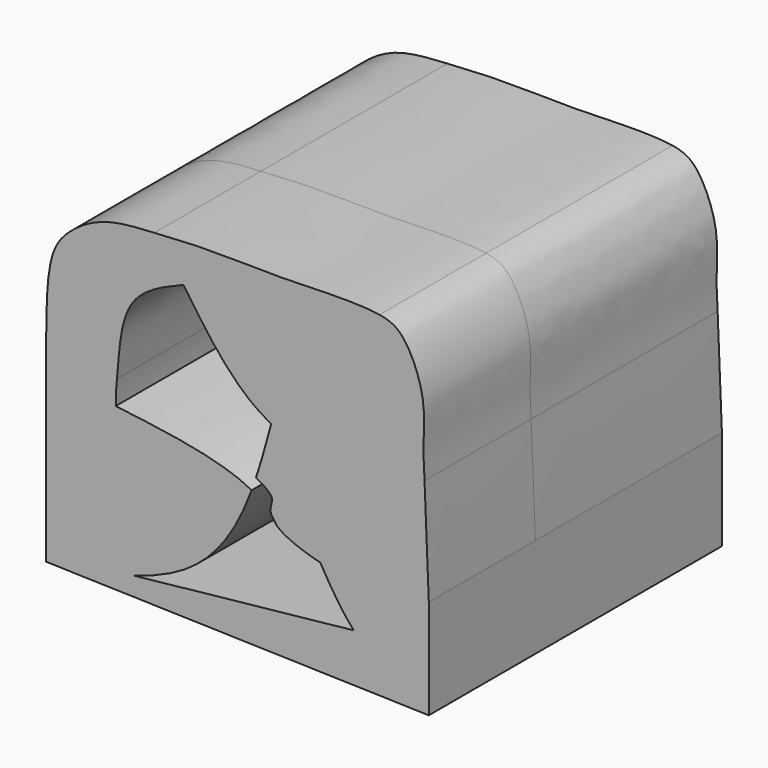
from build123d import *

# Parameters (mm, degrees)
F1_DEPTH = 65.786
F2_DEPTH = 37.592


with BuildPart() as f1:
    # F0 (on Front) → F1 (new body)
    with BuildSketch(Plane.XZ):
        with BuildLine():
            add(Edge.make_bspline(
                [(-63.5240077972, 0), (-56.800894212, -1.0775298684), (-50.0777806268, -2.1550597368), (-43.5278602812, -2.9725744292)],
                knots=[0, 0, 0, 0, 0.1517041989, 0.1517041989, 0.1517041989, 0.1517041989], degree=3))
            add(Edge.make_bspline(
                [(-63.5240077972, 0), (-63.5240077972, -14.8315681088), (-63.5240077972, -38.8086731136), (-63.5240077972, -50.459096132), (-63.5240077972, -54.9028925598)],
                knots=[0, 0, 0, 0, 0.6185720964, 1, 1, 1, 1], degree=3))
            add(Edge.make_bspline(
                [(-38.6864171805, -50.2711780887), (-50.9512119334, -53.9625100963), (-63.4495334183, -54.869292182), (-63.5240077972, -54.9028925598)],
                knots=[0.6463482271, 0.6463482271, 0.6463482271, 0.6463482271, 0.9807009616, 0.9807009616, 0.9807009616, 0.9807009616], degree=3))
            add(Edge.make_bspline(
                [(-5.5222542955, -18.2656030645), (-9.6177271454, -29.334625985), (-17.4503709129, -42.4788636865), (-34.347240688, -48.9652172963), (-38.6864171805, -50.2711780887)],
                knots=[0.1825956876, 0.1825956876, 0.1825956876, 0.1825956876, 0.5280571708, 0.6463482271, 0.6463482271, 0.6463482271, 0.6463482271], degree=3))
            add(Edge.make_bspline(
                [(-5.5222542955, -18.2656030645), (-14.3615559782, -13.5084226746), (-29.1116867734, -11.6697593601), (-43.8618175685, -9.8310960457)],
                knots=[0.536277576, 0.536277576, 0.536277576, 0.536277576, 1, 1, 1, 1], degree=3))
            add(Edge.make_bspline(
                [(-43.5278602812, -2.9725744292), (-43.7574319507, -5.4534811837), (-43.9319764374, -7.5593468165), (-43.8618175685, -9.8310960457)],
                knots=[0.364256955, 0.364256955, 0.364256955, 0.364256955, 0.454666135, 0.454666135, 0.454666135, 0.454666135], degree=3))
        make_face()
        with BuildLine():
            add(Edge.make_bspline(
                [(30.5520221591, 37.0556712151), (34.0105628024, 36.4734212431), (38.1054530927, 33.9530063414), (43.8199870431, 20.7878269574), (42.6933877746, 8.671351149), (43.0629264411, 3.7159273768), (43.2568266988, 0)],
                knots=[0.624432363, 0.624432363, 0.624432363, 0.624432363, 0.6822121522, 0.7571029707, 0.827315679, 0.8883884684, 0.8883884684, 0.8883884684, 0.8883884684], degree=3))
            add(Edge.make_bspline(
                [(13.8594305388, 10.8592628278), (20.3273577037, 18.2346283086), (25.4396899314, 27.6451497618), (30.5520221591, 37.0556712151)],
                knots=[0.7125110381, 0.7125110381, 0.7125110381, 0.7125110381, 1, 1, 1, 1], degree=3))
            add(Edge.make_bspline(
                [(13.8594305388, 10.8592628278), (17.5604882015, 6.5582793426), (21.2565043667, 2.2290147137), (23.9242081779, -3.1279210775)],
                knots=[0, 0, 0, 0, 0.1597565298, 0.1597565298, 0.1597565298, 0.1597565298], degree=3))
            add(Edge.make_bspline(
                [(43.2568266988, 0), (36.7271959027, -1.2648272998), (30.1975651067, -2.5296545995), (23.9242081779, -3.1279210775)],
                knots=[0, 0, 0, 0, 0.1699095992, 0.1699095992, 0.1699095992, 0.1699095992], degree=3))
        make_face()
        with BuildLine():
            add(Edge.make_bspline(
                [(-32.9719856381, 36.7531776428), (-29.0195790904, 36.9869114892), (-21.8300737753, 37.5502432541), (-4.4364884364, 37.370612376), (5.8593016392, 37.152577587), (24.5712134077, 38.0625484176), (30.5520221591, 37.0556712151)],
                knots=[0.3023646182, 0.3023646182, 0.3023646182, 0.3023646182, 0.3717078691, 0.4543133623, 0.524514535, 0.624432363, 0.624432363, 0.624432363, 0.624432363], degree=3))
            add(Edge.make_bspline(
                [(-24.8046126217, 26.4683365822), (-28.1533623745, 31.1750804496), (-30.5626740063, 33.9641290462), (-32.9719856381, 36.7531776428)],
                knots=[0.7766252382, 0.7766252382, 0.7766252382, 0.7766252382, 1, 1, 1, 1], degree=3))
            add(Edge.make_bspline(
                [(0, 0), (-11.0790603922, 5.5270215272), (-19.2392119365, 18.6460394629), (-24.8046126217, 26.4683365822)],
                knots=[0.4053911526, 0.4053911526, 0.4053911526, 0.4053911526, 0.7766252382, 0.7766252382, 0.7766252382, 0.7766252382], degree=3))
            add(Edge.make_bspline(
                [(0, 0), (-1.3505629892, 10.3087183451), (-3.9277431014, 29.9164532393), (8.1573168133, 16.967743401), (13.8594305388, 10.8592628278)],
                knots=[0, 0, 0, 0, 0.5264929724, 1, 1, 1, 1], degree=3))
            add(Edge.make_bspline(
                [(13.8594305388, 10.8592628278), (20.3273577037, 18.2346283086), (25.4396899314, 27.6451497618), (30.5520221591, 37.0556712151)],
                knots=[0.7125110381, 0.7125110381, 0.7125110381, 0.7125110381, 1, 1, 1, 1], degree=3))
        make_face()
        with BuildLine():
            add(Edge.make_bspline(
                [(0, 0), (-1.3505629892, 10.3087183451), (-3.9277431014, 29.9164532393), (8.1573168133, 16.967743401), (13.8594305388, 10.8592628278)],
                knots=[0, 0, 0, 0, 0.5264929724, 1, 1, 1, 1], degree=3))
            add(Edge.make_bspline(
                [(0, 0), (5.3503012941, 2.523067269), (9.8635631765, 6.302782605), (13.8594305388, 10.8592628278)],
                knots=[0.5349011592, 0.5349011592, 0.5349011592, 0.5349011592, 0.7125110381, 0.7125110381, 0.7125110381, 0.7125110381], degree=3))
        make_face()
        with BuildLine():
            add(Edge.make_bspline(
                [(0, 0), (5.3503012941, 2.523067269), (9.8635631765, 6.302782605), (13.8594305388, 10.8592628278)],
                knots=[0.5349011592, 0.5349011592, 0.5349011592, 0.5349011592, 0.7125110381, 0.7125110381, 0.7125110381, 0.7125110381], degree=3))
            add(Edge.make_bspline(
                [(23.9242081779, -3.1279210775), (15.2298210333, -3.9570721102), (7.0276799799, -3.5059054793), (0, 0)],
                knots=[0.1699095992, 0.1699095992, 0.1699095992, 0.1699095992, 0.4053911526, 0.4053911526, 0.4053911526, 0.4053911526], degree=3))
            add(Edge.make_bspline(
                [(13.8594305388, 10.8592628278), (17.5604882015, 6.5582793426), (21.2565043667, 2.2290147137), (23.9242081779, -3.1279210775)],
                knots=[0, 0, 0, 0, 0.1597565298, 0.1597565298, 0.1597565298, 0.1597565298], degree=3))
        make_face()
        with BuildLine():
            add(Edge.make_bspline(
                [(23.9242081779, -3.1279210775), (15.2298210333, -3.9570721102), (7.0276799799, -3.5059054793), (0, 0)],
                knots=[0.1699095992, 0.1699095992, 0.1699095992, 0.1699095992, 0.4053911526, 0.4053911526, 0.4053911526, 0.4053911526], degree=3))
            add(Edge.make_bspline(
                [(0, 0), (4.4728324678, -10.5492547403), (8.9456649356, -21.0985094806), (13.8594305239, -29.9524251855)],
                knots=[0, 0, 0, 0, 0.3636574997, 0.3636574997, 0.3636574997, 0.3636574997], degree=3))
            add(Edge.make_bspline(
                [(23.9242081779, -3.1279210775), (26.6204532145, -8.5421696451), (29.5766972297, -20.153001473), (21.810722237, -31.3197789457), (16.7217291382, -30.6506424008), (13.8594305388, -29.9524252122)],
                knots=[0.1597565298, 0.1597565298, 0.1597565298, 0.1597565298, 0.3212222626, 0.4497849367, 0.5538859787, 0.5538859787, 0.5538859787, 0.5538859787], degree=3))
        make_face()
        with BuildLine():
            add(Edge.make_bspline(
                [(0, 0), (4.4728324678, -10.5492547403), (8.9456649356, -21.0985094806), (13.8594305239, -29.9524251855)],
                knots=[0, 0, 0, 0, 0.3636574997, 0.3636574997, 0.3636574997, 0.3636574997], degree=3))
            add(Edge.make_bspline(
                [(0, 0), (-1.3539150879, -5.0062615134), (-2.7078301758, -10.0125230268), (-4.316626864, -14.8315680972)],
                knots=[0, 0, 0, 0, 0.1472607818, 0.1472607818, 0.1472607818, 0.1472607818], degree=3))
            add(Edge.make_bspline(
                [(0, -22.5358977914), (-0.2635636531, -21.7047236316), (-0.1272346241, -20.0889351399), (0.9365763808, -17.7222891685), (-3.3889358906, -15.1105107507), (-4.3166268678, -14.8315681088)],
                knots=[0.766461406, 0.766461406, 0.766461406, 0.766461406, 0.8263295038, 0.8829450572, 0.9717632395, 0.9717632395, 0.9717632395, 0.9717632395], degree=3))
            add(Edge.make_bspline(
                [(1.488152394, -24.70578484), (1.0691570646, -23.9444424302), (0.5763910158, -23.2195248774), (0, -22.5358977914)],
                knots=[0.3684861738, 0.3684861738, 0.3684861738, 0.3684861738, 0.4177083301, 0.4177083301, 0.4177083301, 0.4177083301], degree=3))
            add(Edge.make_bspline(
                [(13.8594305388, -29.9524252122), (10.2585116388, -29.0740320666), (4.7263466302, -27.2293564363), (1.9133329744, -25.0987912775), (1.488152394, -24.70578484)],
                knots=[0.5538859787, 0.5538859787, 0.5538859787, 0.5538859787, 0.6848504454, 0.7139186659, 0.7139186659, 0.7139186659, 0.7139186659], degree=3))
        make_face()
        with BuildLine():
            add(Edge.make_bspline(
                [(43.2568266988, 0), (43.6111826237, -6.7909186818), (44.038995531, -18.2933515925), (44.4668084383, -29.7957845032)],
                knots=[0.8883884684, 0.8883884684, 0.8883884684, 0.8883884684, 1, 1, 1, 1], degree=3))
            add(Edge.make_bspline(
                [(43.2568266988, 0), (36.7271959027, -1.2648272998), (30.1975651067, -2.5296545995), (23.9242081779, -3.1279210775)],
                knots=[0, 0, 0, 0, 0.1699095992, 0.1699095992, 0.1699095992, 0.1699095992], degree=3))
            add(Edge.make_bspline(
                [(23.9242081779, -3.1279210775), (26.6204532145, -8.5421696451), (29.5766972297, -20.153001473), (21.810722237, -31.3197789457), (16.7217291382, -30.6506424008), (13.8594305388, -29.9524252122)],
                knots=[0.1597565298, 0.1597565298, 0.1597565298, 0.1597565298, 0.3212222626, 0.4497849367, 0.5538859787, 0.5538859787, 0.5538859787, 0.5538859787], degree=3))
            add(Edge.make_bspline(
                [(13.8594305239, -29.9524251855), (16.8125078822, -35.2734559774), (19.9248403959, -39.9821683267), (23.2921373099, -43.7105707824)],
                knots=[0.3636574997, 0.3636574997, 0.3636574997, 0.3636574997, 0.58220857, 0.58220857, 0.58220857, 0.58220857], degree=3))
            add(Edge.make_bspline(
                [(23.2921373099, -43.7105707824), (29.7292039017, -50.8379419353), (37.09800617, -54.3828925593), (44.4668084383, -57.9278431833)],
                knots=[0.58220857, 0.58220857, 0.58220857, 0.58220857, 1, 1, 1, 1], degree=3))
            add(Edge.make_bspline(
                [(44.4668084383, -29.7957845032), (44.4668084383, -39.1731373966), (44.4668084383, -48.5504902899), (44.4668084383, -57.9278431833)],
                knots=[0, 0, 0, 0, 28.1320586801, 28.1320586801, 28.1320586801, 28.1320586801], degree=3))
        make_face()
        with BuildLine():
            add(Edge.make_bspline(
                [(-63.5240077972, 0), (-63.4541196718, 8.3226000217), (-63.3391779129, 22.0103943304), (-56.9568040639, 29.8479836401), (-47.1288987651, 36.0612304876), (-37.335938301, 36.4951061542), (-32.9719856381, 36.7531776428)],
                knots=[0, 0, 0, 0, 0.095878703, 0.1576872566, 0.2258009701, 0.3023646182, 0.3023646182, 0.3023646182, 0.3023646182], degree=3))
            add(Edge.make_bspline(
                [(-63.5240077972, 0), (-56.800894212, -1.0775298684), (-50.0777806268, -2.1550597368), (-43.5278602812, -2.9725744292)],
                knots=[0, 0, 0, 0, 0.1517041989, 0.1517041989, 0.1517041989, 0.1517041989], degree=3))
            add(Edge.make_bspline(
                [(-24.8046126217, 26.4683365822), (-30.5304064505, 24.1328709252), (-42.0237334945, 19.4449147399), (-42.8894476385, 3.7449684225), (-43.4419108928, -2.043747198), (-43.5278602812, -2.9725744292)],
                knots=[0, 0, 0, 0, 0.1646043618, 0.330408642, 0.364256955, 0.364256955, 0.364256955, 0.364256955], degree=3))
            add(Edge.make_bspline(
                [(-24.8046126217, 26.4683365822), (-28.1533623745, 31.1750804496), (-30.5626740063, 33.9641290462), (-32.9719856381, 36.7531776428)],
                knots=[0.7766252382, 0.7766252382, 0.7766252382, 0.7766252382, 1, 1, 1, 1], degree=3))
        make_face()
        with BuildLine():
            add(Edge.make_bspline(
                [(-38.6864171805, -50.2711780887), (-50.9512119334, -53.9625100963), (-63.4495334183, -54.869292182), (-63.5240077972, -54.9028925598)],
                knots=[0.6463482271, 0.6463482271, 0.6463482271, 0.6463482271, 0.9807009616, 0.9807009616, 0.9807009616, 0.9807009616], degree=3))
            add(Edge.make_bspline(
                [(-63.5240077972, -54.9028925598), (-63.5283065026, -54.9048319935), (-63.4912130872, -54.9038622766), (-63.4541196718, -54.9028925598)],
                knots=[0.9807009616, 0.9807009616, 0.9807009616, 0.9807009616, 1, 1, 1, 1], degree=3))
            add(Edge.make_bspline(
                [(-63.4541196718, -54.9028925598), (-27.4804769685, -55.9112094343), (8.4931657349, -56.9195263088), (44.4668084383, -57.9278431833)],
                knots=[0, 0, 0, 0, 107.9633134469, 107.9633134469, 107.9633134469, 107.9633134469], degree=3))
            add(Edge.make_bspline(
                [(23.2921373099, -43.7105707824), (29.7292039017, -50.8379419353), (37.09800617, -54.3828925593), (44.4668084383, -57.9278431833)],
                knots=[0.58220857, 0.58220857, 0.58220857, 0.58220857, 1, 1, 1, 1], degree=3))
            add(Edge.make_bspline(
                [(-38.6864171805, -50.2711780887), (-18.0238019664, -48.094599226), (2.6295220958, -45.8871496451), (23.2921373099, -43.7105707824)],
                knots=[0, 0, 0, 0, 62.3248167662, 62.3248167662, 62.3248167662, 62.3248167662], degree=3))
        make_face()
    extrude(amount=-F1_DEPTH)

    # F0 (on Front) + F1_face (on face) + F1_face1 (on face) → F2 (join)
    with BuildSketch(Plane.XZ):
        with BuildLine():
            add(Edge.make_bspline(
                [(-63.5240077972, 0), (-63.4541196718, 8.3226000217), (-63.3391779129, 22.0103943304), (-56.9568040639, 29.8479836401), (-47.1288987651, 36.0612304876), (-37.335938301, 36.4951061542), (-32.9719856381, 36.7531776428)],
                knots=[0, 0, 0, 0, 0.095878703, 0.1576872566, 0.2258009701, 0.3023646182, 0.3023646182, 0.3023646182, 0.3023646182], degree=3))
            add(Edge.make_bspline(
                [(-63.5240077972, 0), (-56.800894212, -1.0775298684), (-50.0777806268, -2.1550597368), (-43.5278602812, -2.9725744292)],
                knots=[0, 0, 0, 0, 0.1517041989, 0.1517041989, 0.1517041989, 0.1517041989], degree=3))
            add(Edge.make_bspline(
                [(-24.8046126217, 26.4683365822), (-30.5304064505, 24.1328709252), (-42.0237334945, 19.4449147399), (-42.8894476385, 3.7449684225), (-43.4419108928, -2.043747198), (-43.5278602812, -2.9725744292)],
                knots=[0, 0, 0, 0, 0.1646043618, 0.330408642, 0.364256955, 0.364256955, 0.364256955, 0.364256955], degree=3))
            add(Edge.make_bspline(
                [(-24.8046126217, 26.4683365822), (-28.1533623745, 31.1750804496), (-30.5626740063, 33.9641290462), (-32.9719856381, 36.7531776428)],
                knots=[0.7766252382, 0.7766252382, 0.7766252382, 0.7766252382, 1, 1, 1, 1], degree=3))
        make_face()
        with BuildLine():
            add(Edge.make_bspline(
                [(30.5520221591, 37.0556712151), (34.0105628024, 36.4734212431), (38.1054530927, 33.9530063414), (43.8199870431, 20.7878269574), (42.6933877746, 8.671351149), (43.0629264411, 3.7159273768), (43.2568266988, 0)],
                knots=[0.624432363, 0.624432363, 0.624432363, 0.624432363, 0.6822121522, 0.7571029707, 0.827315679, 0.8883884684, 0.8883884684, 0.8883884684, 0.8883884684], degree=3))
            add(Edge.make_bspline(
                [(13.8594305388, 10.8592628278), (20.3273577037, 18.2346283086), (25.4396899314, 27.6451497618), (30.5520221591, 37.0556712151)],
                knots=[0.7125110381, 0.7125110381, 0.7125110381, 0.7125110381, 1, 1, 1, 1], degree=3))
            add(Edge.make_bspline(
                [(13.8594305388, 10.8592628278), (17.5604882015, 6.5582793426), (21.2565043667, 2.2290147137), (23.9242081779, -3.1279210775)],
                knots=[0, 0, 0, 0, 0.1597565298, 0.1597565298, 0.1597565298, 0.1597565298], degree=3))
            add(Edge.make_bspline(
                [(43.2568266988, 0), (36.7271959027, -1.2648272998), (30.1975651067, -2.5296545995), (23.9242081779, -3.1279210775)],
                knots=[0, 0, 0, 0, 0.1699095992, 0.1699095992, 0.1699095992, 0.1699095992], degree=3))
        make_face()
        with BuildLine():
            add(Edge.make_bspline(
                [(-38.6864171805, -50.2711780887), (-50.9512119334, -53.9625100963), (-63.4495334183, -54.869292182), (-63.5240077972, -54.9028925598)],
                knots=[0.6463482271, 0.6463482271, 0.6463482271, 0.6463482271, 0.9807009616, 0.9807009616, 0.9807009616, 0.9807009616], degree=3))
            add(Edge.make_bspline(
                [(-63.5240077972, -54.9028925598), (-63.5283065026, -54.9048319935), (-63.4912130872, -54.9038622766), (-63.4541196718, -54.9028925598)],
                knots=[0.9807009616, 0.9807009616, 0.9807009616, 0.9807009616, 1, 1, 1, 1], degree=3))
            add(Edge.make_bspline(
                [(-63.4541196718, -54.9028925598), (-27.4804769685, -55.9112094343), (8.4931657349, -56.9195263088), (44.4668084383, -57.9278431833)],
                knots=[0, 0, 0, 0, 107.9633134469, 107.9633134469, 107.9633134469, 107.9633134469], degree=3))
            add(Edge.make_bspline(
                [(23.2921373099, -43.7105707824), (29.7292039017, -50.8379419353), (37.09800617, -54.3828925593), (44.4668084383, -57.9278431833)],
                knots=[0.58220857, 0.58220857, 0.58220857, 0.58220857, 1, 1, 1, 1], degree=3))
            add(Edge.make_bspline(
                [(-38.6864171805, -50.2711780887), (-18.0238019664, -48.094599226), (2.6295220958, -45.8871496451), (23.2921373099, -43.7105707824)],
                knots=[0, 0, 0, 0, 62.3248167662, 62.3248167662, 62.3248167662, 62.3248167662], degree=3))
        make_face()
        with BuildLine():
            add(Edge.make_bspline(
                [(-32.9719856381, 36.7531776428), (-29.0195790904, 36.9869114892), (-21.8300737753, 37.5502432541), (-4.4364884364, 37.370612376), (5.8593016392, 37.152577587), (24.5712134077, 38.0625484176), (30.5520221591, 37.0556712151)],
                knots=[0.3023646182, 0.3023646182, 0.3023646182, 0.3023646182, 0.3717078691, 0.4543133623, 0.524514535, 0.624432363, 0.624432363, 0.624432363, 0.624432363], degree=3))
            add(Edge.make_bspline(
                [(-24.8046126217, 26.4683365822), (-28.1533623745, 31.1750804496), (-30.5626740063, 33.9641290462), (-32.9719856381, 36.7531776428)],
                knots=[0.7766252382, 0.7766252382, 0.7766252382, 0.7766252382, 1, 1, 1, 1], degree=3))
            add(Edge.make_bspline(
                [(0, 0), (-11.0790603922, 5.5270215272), (-19.2392119365, 18.6460394629), (-24.8046126217, 26.4683365822)],
                knots=[0.4053911526, 0.4053911526, 0.4053911526, 0.4053911526, 0.7766252382, 0.7766252382, 0.7766252382, 0.7766252382], degree=3))
            add(Edge.make_bspline(
                [(0, 0), (-1.3505629892, 10.3087183451), (-3.9277431014, 29.9164532393), (8.1573168133, 16.967743401), (13.8594305388, 10.8592628278)],
                knots=[0, 0, 0, 0, 0.5264929724, 1, 1, 1, 1], degree=3))
            add(Edge.make_bspline(
                [(13.8594305388, 10.8592628278), (20.3273577037, 18.2346283086), (25.4396899314, 27.6451497618), (30.5520221591, 37.0556712151)],
                knots=[0.7125110381, 0.7125110381, 0.7125110381, 0.7125110381, 1, 1, 1, 1], degree=3))
        make_face()
        with BuildLine():
            add(Edge.make_bspline(
                [(43.2568266988, 0), (43.6111826237, -6.7909186818), (44.038995531, -18.2933515925), (44.4668084383, -29.7957845032)],
                knots=[0.8883884684, 0.8883884684, 0.8883884684, 0.8883884684, 1, 1, 1, 1], degree=3))
            add(Edge.make_bspline(
                [(43.2568266988, 0), (36.7271959027, -1.2648272998), (30.1975651067, -2.5296545995), (23.9242081779, -3.1279210775)],
                knots=[0, 0, 0, 0, 0.1699095992, 0.1699095992, 0.1699095992, 0.1699095992], degree=3))
            add(Edge.make_bspline(
                [(23.9242081779, -3.1279210775), (26.6204532145, -8.5421696451), (29.5766972297, -20.153001473), (21.810722237, -31.3197789457), (16.7217291382, -30.6506424008), (13.8594305388, -29.9524252122)],
                knots=[0.1597565298, 0.1597565298, 0.1597565298, 0.1597565298, 0.3212222626, 0.4497849367, 0.5538859787, 0.5538859787, 0.5538859787, 0.5538859787], degree=3))
            add(Edge.make_bspline(
                [(13.8594305239, -29.9524251855), (16.8125078822, -35.2734559774), (19.9248403959, -39.9821683267), (23.2921373099, -43.7105707824)],
                knots=[0.3636574997, 0.3636574997, 0.3636574997, 0.3636574997, 0.58220857, 0.58220857, 0.58220857, 0.58220857], degree=3))
            add(Edge.make_bspline(
                [(23.2921373099, -43.7105707824), (29.7292039017, -50.8379419353), (37.09800617, -54.3828925593), (44.4668084383, -57.9278431833)],
                knots=[0.58220857, 0.58220857, 0.58220857, 0.58220857, 1, 1, 1, 1], degree=3))
            add(Edge.make_bspline(
                [(44.4668084383, -29.7957845032), (44.4668084383, -39.1731373966), (44.4668084383, -48.5504902899), (44.4668084383, -57.9278431833)],
                knots=[0, 0, 0, 0, 28.1320586801, 28.1320586801, 28.1320586801, 28.1320586801], degree=3))
        make_face()
        with BuildLine():
            add(Edge.make_bspline(
                [(-63.5240077972, 0), (-56.800894212, -1.0775298684), (-50.0777806268, -2.1550597368), (-43.5278602812, -2.9725744292)],
                knots=[0, 0, 0, 0, 0.1517041989, 0.1517041989, 0.1517041989, 0.1517041989], degree=3))
            add(Edge.make_bspline(
                [(-63.5240077972, 0), (-63.5240077972, -14.8315681088), (-63.5240077972, -38.8086731136), (-63.5240077972, -50.459096132), (-63.5240077972, -54.9028925598)],
                knots=[0, 0, 0, 0, 0.6185720964, 1, 1, 1, 1], degree=3))
            add(Edge.make_bspline(
                [(-38.6864171805, -50.2711780887), (-50.9512119334, -53.9625100963), (-63.4495334183, -54.869292182), (-63.5240077972, -54.9028925598)],
                knots=[0.6463482271, 0.6463482271, 0.6463482271, 0.6463482271, 0.9807009616, 0.9807009616, 0.9807009616, 0.9807009616], degree=3))
            add(Edge.make_bspline(
                [(-5.5222542955, -18.2656030645), (-9.6177271454, -29.334625985), (-17.4503709129, -42.4788636865), (-34.347240688, -48.9652172963), (-38.6864171805, -50.2711780887)],
                knots=[0.1825956876, 0.1825956876, 0.1825956876, 0.1825956876, 0.5280571708, 0.6463482271, 0.6463482271, 0.6463482271, 0.6463482271], degree=3))
            add(Edge.make_bspline(
                [(-5.5222542955, -18.2656030645), (-14.3615559782, -13.5084226746), (-29.1116867734, -11.6697593601), (-43.8618175685, -9.8310960457)],
                knots=[0.536277576, 0.536277576, 0.536277576, 0.536277576, 1, 1, 1, 1], degree=3))
            add(Edge.make_bspline(
                [(-43.5278602812, -2.9725744292), (-43.7574319507, -5.4534811837), (-43.9319764374, -7.5593468165), (-43.8618175685, -9.8310960457)],
                knots=[0.364256955, 0.364256955, 0.364256955, 0.364256955, 0.454666135, 0.454666135, 0.454666135, 0.454666135], degree=3))
        make_face()
    with BuildSketch(Plane(origin=(-7.6226899771, 0, -10.0369627759), x_dir=(1, 0, 0), z_dir=(0, -1, 0))):
        with BuildLine():
            add(Edge.make_bspline(
                [(-55.9013178202, 10.0369627759), (-55.9013178202, -4.7946053329), (-55.9013178202, -28.7717103377), (-55.9013178202, -40.4221333561), (-55.9013178202, -44.8659297839)],
                knots=[0, 0, 0, 0, 0.6185720964, 1, 1, 1, 1], degree=3))
            add(Edge.make_bspline(
                [(-55.9013178202, -44.8659297839), (-55.9056165255, -44.8678692176), (-55.8685231102, -44.8668995008), (-55.8314296948, -44.8659297839)],
                knots=[0.9807009616, 0.9807009616, 0.9807009616, 0.9807009616, 1, 1, 1, 1], degree=3))
            add(Edge.make_bspline(
                [(-55.8314296948, -44.8659297839), (-19.8577869914, -45.8742466584), (16.115855712, -46.8825635329), (52.0894984154, -47.8908804074)],
                knots=[0, 0, 0, 0, 107.9633134469, 107.9633134469, 107.9633134469, 107.9633134469], degree=3))
            add(Edge.make_bspline(
                [(52.0894984154, -19.7588217273), (52.0894984154, -29.1361746207), (52.0894984154, -38.513527514), (52.0894984154, -47.8908804074)],
                knots=[0, 0, 0, 0, 28.1320586801, 28.1320586801, 28.1320586801, 28.1320586801], degree=3))
            add(Edge.make_bspline(
                [(52.0894984154, -19.7588217273), (51.6616855081, -8.2563888166), (50.9997773673, 9.5400681217), (50.3160777517, 18.7083139249), (51.4426770202, 30.8247897333), (45.7281430698, 43.9899691172), (38.5492799946, 48.4085767452), (13.4819916163, 47.1895403629), (3.1862015407, 47.4075751518), (-14.2073837983, 47.58720603), (-25.0195235656, 46.7400237121), (-39.506208788, 46.0981932634), (-49.3341140868, 39.884946416), (-55.7164879359, 32.0473571063), (-55.8314296948, 18.3595627976), (-55.9013178202, 10.0369627759)],
                knots=[0.8883884684, 0.8883884684, 0.8883884684, 0.8883884684, 1, 1.0610727893, 1.1312854977, 1.2061763162, 1.2639561054, 1.3638739333, 1.434075106, 1.5166805993, 1.5860238501, 1.6625874983, 1.7307012118, 1.7925097654, 1.8883884684, 1.8883884684, 1.8883884684, 1.8883884684], degree=3))
        make_face()
        with BuildLine():
            add(Edge.make_bspline(
                [(-31.0637272034, -40.2342153128), (-26.7245507109, -38.9282545204), (-9.8276809358, -32.4419009106), (-1.9950371683, -19.2976632091), (2.1004356815, -8.2286402886)],
                knots=[0.9807009616, 0.9807009616, 0.9807009616, 0.9807009616, 1.0989920179, 1.4444535011, 1.4444535011, 1.4444535011, 1.4444535011], degree=3))
            add(Edge.make_bspline(
                [(2.1004356815, -8.2286402886), (-6.7388660012, -3.4714598987), (-21.4889967963, -1.6327965842), (-36.2391275915, 0.2058667302)],
                knots=[0.536277576, 0.536277576, 0.536277576, 0.536277576, 1, 1, 1, 1], degree=3))
            add(Edge.make_bspline(
                [(-36.2391275915, 0.2058667302), (-36.3355532548, 3.3281366583), (-35.4816293471, 9.8851784973), (-34.4010435174, 29.4818775158), (-22.9077164735, 34.1698337011), (-17.1819226446, 36.5052993581)],
                knots=[0.364256955, 0.364256955, 0.364256955, 0.364256955, 0.488514448, 0.6543187282, 0.81892309, 0.81892309, 0.81892309, 0.81892309], degree=3))
            add(Edge.make_bspline(
                [(-17.1819226446, 36.5052993581), (-11.6165219594, 28.6830022388), (-3.4563704151, 15.563984303), (7.6226899771, 10.0369627759)],
                knots=[1, 1, 1, 1, 1.3712340856, 1.3712340856, 1.3712340856, 1.3712340856], degree=3))
            add(Edge.make_bspline(
                [(7.6226899771, 10.0369627759), (6.2687748892, 5.0307012625), (4.9148598012, 0.0244397491), (3.3060631131, -4.7946053213)],
                knots=[0, 0, 0, 0, 0.1472607818, 0.1472607818, 0.1472607818, 0.1472607818], degree=3))
            add(Edge.make_bspline(
                [(7.6226899771, -12.4989350155), (7.359126324, -11.6677608557), (7.4954553529, -10.051972364), (8.5592663579, -7.6853263926), (4.2337540865, -5.0735479748), (3.3060631093, -4.7946053329)],
                knots=[0.766461406, 0.766461406, 0.766461406, 0.766461406, 0.8263295038, 0.8829450572, 0.9717632395, 0.9717632395, 0.9717632395, 0.9717632395], degree=3))
            add(Edge.make_bspline(
                [(9.110842371, -14.6688220641), (8.6918470417, -13.9074796543), (8.1990809928, -13.1825621015), (7.6226899771, -12.4989350155)],
                knots=[0.3684861738, 0.3684861738, 0.3684861738, 0.3684861738, 0.4177083301, 0.4177083301, 0.4177083301, 0.4177083301], degree=3))
            add(Edge.make_bspline(
                [(9.110842371, -14.6688220641), (9.5360229514, -15.0618285016), (12.3490366073, -17.1923936605), (17.8812016159, -19.0370692907), (21.4821205158, -19.9154624363)],
                knots=[0.5538859787, 0.5538859787, 0.5538859787, 0.5538859787, 0.5829541992, 0.7139186659, 0.7139186659, 0.7139186659, 0.7139186659], degree=3))
            add(Edge.make_bspline(
                [(21.482120501, -19.9154624096), (24.4351978592, -25.2364932015), (27.5475303729, -29.9452055508), (30.914827287, -33.6736080065)],
                knots=[0.3636574997, 0.3636574997, 0.3636574997, 0.3636574997, 0.58220857, 0.58220857, 0.58220857, 0.58220857], degree=3))
            add(Edge.make_bspline(
                [(-31.0637272034, -40.2342153128), (-10.4011119893, -38.0576364501), (10.2522120729, -35.8501868692), (30.914827287, -33.6736080065)],
                knots=[0, 0, 0, 0, 62.3248167662, 62.3248167662, 62.3248167662, 62.3248167662], degree=3))
        make_face(mode=Mode.SUBTRACT)
    with BuildSketch(Plane(origin=(-7.6226899771, 65.786, -10.0369627759), x_dir=(1, 0, 0), z_dir=(0, 1, 0))):
        with BuildLine():
            add(Edge.make_bspline(
                [(-55.9013178202, -10.0369627759), (-55.9013178202, 4.7946053329), (-55.9013178202, 28.7717103377), (-55.9013178202, 40.4221333561), (-55.9013178202, 44.8659297839)],
                knots=[0, 0, 0, 0, 0.6185720964, 1, 1, 1, 1], degree=3))
            add(Edge.make_bspline(
                [(52.0894984154, 19.7588217273), (51.6616855081, 8.2563888166), (50.9997773673, -9.5400681217), (50.3160777517, -18.7083139249), (51.4426770202, -30.8247897333), (45.7281430698, -43.9899691172), (38.5492799946, -48.4085767452), (13.4819916163, -47.1895403629), (3.1862015407, -47.4075751518), (-14.2073837983, -47.58720603), (-25.0195235656, -46.7400237121), (-39.506208788, -46.0981932634), (-49.3341140868, -39.884946416), (-55.7164879359, -32.0473571063), (-55.8314296948, -18.3595627976), (-55.9013178202, -10.0369627759)],
                knots=[0.8883884684, 0.8883884684, 0.8883884684, 0.8883884684, 1, 1.0610727893, 1.1312854977, 1.2061763162, 1.2639561054, 1.3638739333, 1.434075106, 1.5166805993, 1.5860238501, 1.6625874983, 1.7307012118, 1.7925097654, 1.8883884684, 1.8883884684, 1.8883884684, 1.8883884684], degree=3))
            add(Edge.make_bspline(
                [(52.0894984154, 19.7588217273), (52.0894984154, 29.1361746207), (52.0894984154, 38.513527514), (52.0894984154, 47.8908804074)],
                knots=[0, 0, 0, 0, 28.1320586801, 28.1320586801, 28.1320586801, 28.1320586801], degree=3))
            add(Edge.make_bspline(
                [(-55.8314296948, 44.8659297839), (-19.8577869914, 45.8742466584), (16.115855712, 46.8825635329), (52.0894984154, 47.8908804074)],
                knots=[0, 0, 0, 0, 107.9633134469, 107.9633134469, 107.9633134469, 107.9633134469], degree=3))
            add(Edge.make_bspline(
                [(-55.9013178202, 44.8659297839), (-55.9056165255, 44.8678692176), (-55.8685231102, 44.8668995008), (-55.8314296948, 44.8659297839)],
                knots=[0.9807009616, 0.9807009616, 0.9807009616, 0.9807009616, 1, 1, 1, 1], degree=3))
        make_face()
        with BuildLine():
            add(Edge.make_bspline(
                [(-31.0637272034, 40.2342153128), (-26.7245507109, 38.9282545204), (-9.8276809358, 32.4419009106), (-1.9950371683, 19.2976632091), (2.1004356815, 8.2286402886)],
                knots=[0.9807009616, 0.9807009616, 0.9807009616, 0.9807009616, 1.0989920179, 1.4444535011, 1.4444535011, 1.4444535011, 1.4444535011], degree=3))
            add(Edge.make_bspline(
                [(-31.0637272034, 40.2342153128), (-10.4011119893, 38.0576364501), (10.2522120729, 35.8501868692), (30.914827287, 33.6736080065)],
                knots=[0, 0, 0, 0, 62.3248167662, 62.3248167662, 62.3248167662, 62.3248167662], degree=3))
            add(Edge.make_bspline(
                [(21.482120501, 19.9154624096), (24.4351978592, 25.2364932015), (27.5475303729, 29.9452055508), (30.914827287, 33.6736080065)],
                knots=[0.3636574997, 0.3636574997, 0.3636574997, 0.3636574997, 0.58220857, 0.58220857, 0.58220857, 0.58220857], degree=3))
            add(Edge.make_bspline(
                [(9.110842371, 14.6688220641), (9.5360229514, 15.0618285016), (12.3490366073, 17.1923936605), (17.8812016159, 19.0370692907), (21.4821205158, 19.9154624363)],
                knots=[0.5538859787, 0.5538859787, 0.5538859787, 0.5538859787, 0.5829541992, 0.7139186659, 0.7139186659, 0.7139186659, 0.7139186659], degree=3))
            add(Edge.make_bspline(
                [(9.110842371, 14.6688220641), (8.6918470417, 13.9074796543), (8.1990809928, 13.1825621015), (7.6226899771, 12.4989350155)],
                knots=[0.3684861738, 0.3684861738, 0.3684861738, 0.3684861738, 0.4177083301, 0.4177083301, 0.4177083301, 0.4177083301], degree=3))
            add(Edge.make_bspline(
                [(7.6226899771, 12.4989350155), (7.359126324, 11.6677608557), (7.4954553529, 10.051972364), (8.5592663579, 7.6853263926), (4.2337540865, 5.0735479748), (3.3060631093, 4.7946053329)],
                knots=[0.766461406, 0.766461406, 0.766461406, 0.766461406, 0.8263295038, 0.8829450572, 0.9717632395, 0.9717632395, 0.9717632395, 0.9717632395], degree=3))
            add(Edge.make_bspline(
                [(7.6226899771, -10.0369627759), (6.2687748892, -5.0307012625), (4.9148598012, -0.0244397491), (3.3060631131, 4.7946053213)],
                knots=[0, 0, 0, 0, 0.1472607818, 0.1472607818, 0.1472607818, 0.1472607818], degree=3))
            add(Edge.make_bspline(
                [(-17.1819226446, -36.5052993581), (-11.6165219594, -28.6830022388), (-3.4563704151, -15.563984303), (7.6226899771, -10.0369627759)],
                knots=[1, 1, 1, 1, 1.3712340856, 1.3712340856, 1.3712340856, 1.3712340856], degree=3))
            add(Edge.make_bspline(
                [(-36.2391275915, -0.2058667302), (-36.3355532548, -3.3281366583), (-35.4816293471, -9.8851784973), (-34.4010435174, -29.4818775158), (-22.9077164735, -34.1698337011), (-17.1819226446, -36.5052993581)],
                knots=[0.364256955, 0.364256955, 0.364256955, 0.364256955, 0.488514448, 0.6543187282, 0.81892309, 0.81892309, 0.81892309, 0.81892309], degree=3))
            add(Edge.make_bspline(
                [(2.1004356815, 8.2286402886), (-6.7388660012, 3.4714598987), (-21.4889967963, 1.6327965842), (-36.2391275915, -0.2058667302)],
                knots=[0.536277576, 0.536277576, 0.536277576, 0.536277576, 1, 1, 1, 1], degree=3))
        make_face(mode=Mode.SUBTRACT)
    extrude(amount=F2_DEPTH, dir=(0, -1, 0))


solid = f1.part
